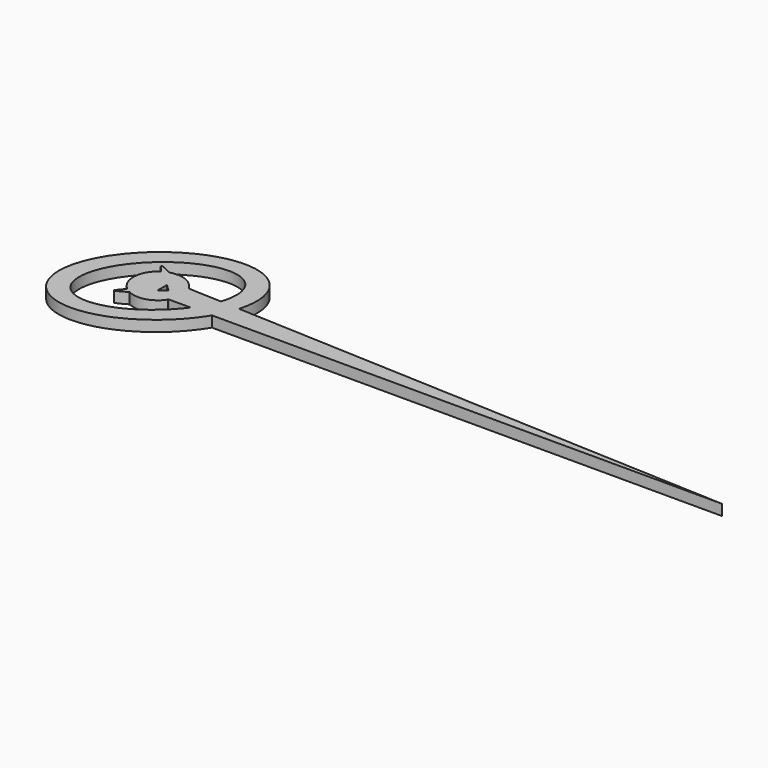
from build123d import *

# Parameters (mm, degrees)
F1_DEPTH = 2.54


# Not quite as in the source:
# - a feature names something its author has since deleted; it is built from what else it names


with BuildPart() as f1:
    # F0 (on Top) → F1 (new body)
    with BuildSketch(Plane.XY):
        with BuildLine():
            ThreePointArc((-75.8652047354, 37.588779241), (-75.1994350162, 37.9605298718), (-74.4903137067, 38.240877547))
            add(Edge.make_bspline(
                [(-75.8652047354, 37.588779241), (-76.604224067, 38.4137884205), (-78.1981423403, 40.1935134784), (-75.778702664, 38.920881298), (-74.4903137067, 38.240877547)],
                knots=[0, 0, 0, 0, 0.4664775591, 1, 1, 1, 1], degree=3))
        make_face()
        with BuildLine():
            add(Edge.make_bspline(
                [(-76.3861294689, 28.3272341561), (-77.2286455281, 27.4100753254), (-78.989872456, 25.4917535729), (-76.5188170846, 26.874194918), (-75.2340137405, 27.5907563812)],
                knots=[0, 0, 0, 0, 0.4793293454, 1, 1, 1, 1], degree=3))
            ThreePointArc((-75.2340137405, 27.5907563812), (-75.8320510764, 27.9246114815), (-76.3861294689, 28.3272341561))
        make_face()
        with BuildLine():
            Line((-59.8411278552, 35.1595323087), (-55.3810254851, 34.9645812086))
            add(Edge.make_bspline(
                [(-55.3810254851, 34.9645812086), (-48.2332464618, 59.6436415888), (-74.8055976533, 47.3367482699), (-101.3779488448, 35.029854951), (-88.5350008625, 19.6094312212)],
                knots=[2.3703033236, 2.3703033236, 2.3703033236, 4.3267443154, 4.3267443154, 6.2831853072, 6.2831853072, 6.2831853072], degree=2, weights=[1, 0.5584995375, 1, 0.5584995375, 1]))
            add(Edge.make_bspline(
                [(-88.5350008625, 19.6094312212), (-74.1070210535, 2.2858726015), (-57.6621755507, 29.8147089779)],
                knots=[0, 0, 0, 2.061745172, 2.061745172, 2.061745172], degree=2, weights=[1, 0.514070582, 1]))
            Line((-57.6621755507, 29.8147089779), (-62.6683754349, 29.8147089779))
            add(Edge.make_bspline(
                [(-60.7383996248, 43.4973761439), (-80.8420671588, 65.9766930493), (-86.1954495571, 28.0236010013), (-91.5488319555, -9.9294910468), (-62.6683754349, 29.8147089779)],
                knots=[0, 0, 0, 2.5317574132, 2.5317574132, 5.0635148264, 5.0635148264, 5.0635148264], degree=2, weights=[1, 0.3002145965, 1, 0.3002145965, 1]))
            add(Edge.make_bspline(
                [(-59.8411278552, 35.1595323087), (-58.0608375325, 40.5034066751), (-60.7383996248, 43.4973761439)],
                knots=[5.4825336434, 5.4825336434, 5.4825336434, 6.2831853072, 6.2831853072, 6.2831853072], degree=2, weights=[1, 0.9209340602, 1]))
        make_face()
        with BuildLine():
            add(Edge.make_bspline(
                [(-57.6621755507, 29.8147089779), (-56.1294482804, 32.3805098074), (-55.3810254851, 34.9645812086)],
                knots=[2.061745172, 2.061745172, 2.061745172, 2.3703033236, 2.3703033236, 2.3703033236], degree=2, weights=[1, 0.9881225704, 1]))
            Line((-55.3810254851, 34.9645812086), (-59.8411278552, 35.1595323087))
            add(Edge.make_bspline(
                [(-62.6683754349, 29.8147089779), (-60.7356522323, 32.4744500905), (-59.8411278552, 35.1595323087)],
                knots=[5.0635148264, 5.0635148264, 5.0635148264, 5.4825336434, 5.4825336434, 5.4825336434], degree=2, weights=[1, 0.9781330657, 1]))
            Line((-62.6683754349, 29.8147089779), (-57.6621755507, 29.8147089779))
        make_face()
        with BuildLine():
            Line((-57.6621755507, 29.8147089779), (62.438044697, 29.8147089779))
            Line((62.438044697, 29.8147089779), (-55.3810254851, 34.9645812086))
            add(Edge.make_bspline(
                [(-57.6621755507, 29.8147089779), (-56.1294482804, 32.3805098074), (-55.3810254851, 34.9645812086)],
                knots=[2.061745172, 2.061745172, 2.061745172, 2.3703033236, 2.3703033236, 2.3703033236], degree=2, weights=[1, 0.9881225704, 1]))
        make_face()
        with BuildLine():
            add(Edge.make_bspline(
                [(-62.6683754349, 29.8147089779), (-60.7356522323, 32.4744500905), (-59.8411278552, 35.1595323087)],
                knots=[5.0635148264, 5.0635148264, 5.0635148264, 5.4825336434, 5.4825336434, 5.4825336434], degree=2, weights=[1, 0.9781330657, 1]))
            Line((-59.8411278552, 35.1595323087), (-67.5292090986, 35.4955783838))
            Line((-67.5292090986, 35.4955783838), (-67.74773377, 35.6220386313))
            ThreePointArc((-67.74773377, 35.6220386313), (-70.6554109693, 38.1250962836), (-74.4903137067, 38.240877547))
            ThreePointArc((-74.4903137067, 38.240877547), (-75.1994350162, 37.9605298718), (-75.8652047354, 37.588779241))
            ThreePointArc((-75.8652047354, 37.588779241), (-78.4749567451, 33.0901448105), (-76.3861294689, 28.3272341561))
            ThreePointArc((-76.3861294689, 28.3272341561), (-75.8320510764, 27.9246114815), (-75.2340137405, 27.5907563812))
            ThreePointArc((-75.2340137405, 27.5907563812), (-71.1447945546, 27.2444669), (-67.8669635062, 29.7137691443))
            Line((-67.8669635062, 29.7137691443), (-67.6427260041, 29.8147089779))
            Line((-67.6427260041, 29.8147089779), (-62.6683754349, 29.8147089779))
        make_face()
        Polygon((-70.1181069016, 32.6280742884), (-71.660593152, 31.267054379), (-71.660593152, 34.0798310935), align=None, mode=Mode.SUBTRACT)
    extrude(amount=-F1_DEPTH)


solid = f1.part
